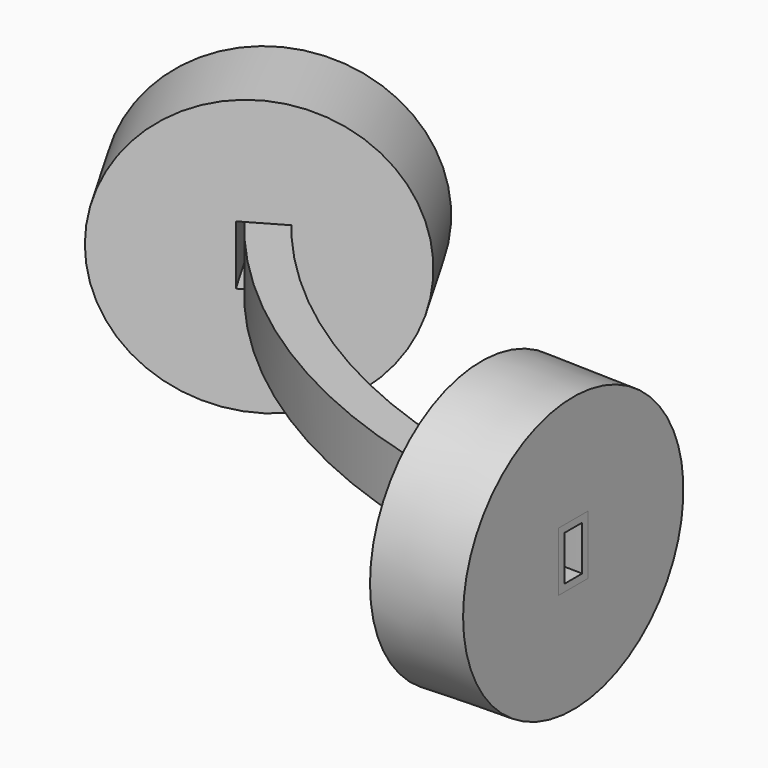
from build123d import *

# Parameters (mm, degrees)
F4_W     = 2.55
F4_H     = 4.1
F4_W_2   = 1.55
F4_H_2   = 3.1
F3_W     = 2.55
F3_H     = 4.1
F3_W_2   = 1.55
F3_H_2   = 3.1
F3_R     = 9.525
F7_DEPTH = 6.35
F4_R     = 9.525
F8_DEPTH = 6.35
F8_TAPER = -1


# Not quite as in the source:
# - a feature of the source that left no trace in its solid (it failed there, or was rolled back) is left out


with BuildPart() as f5:
    # F5: sweep along a path in F0
    with BuildLine(Plane.XY) as f5_path:
        ThreePointArc((-12.7, 21.9970452561), (3.4029547439, 5.8940905122), (25.4, 0))
    # F4 (on line) + F3 (on line) → F5 (sweep)
    with BuildSketch(Plane(origin=(25.4, 0, 0), x_dir=(0, -1, 0), z_dir=(-1, 0, 0))):
        Rectangle(F4_W, F4_H)
        Rectangle(F4_W_2, F4_H_2, mode=Mode.SUBTRACT)
    with BuildSketch(Plane(origin=(-12.7, 21.9970452561, 0), x_dir=(-0.8660254038, -0.5, 0), z_dir=(-0.5, 0.8660254038, 0))):
        Rectangle(F3_W, F3_H)
        Rectangle(F3_W_2, F3_H_2, mode=Mode.SUBTRACT)
    sweep(path=f5_path.line)

    # F4 (on line) → F8 (join)
    with BuildSketch(Plane(origin=(25.4, 0, 0), x_dir=(0, -1, 0), z_dir=(-1, 0, 0))):
        Circle(F4_R)
        Rectangle(F4_W, F4_H, mode=Mode.SUBTRACT)
    extrude(amount=F8_DEPTH, taper=F8_TAPER)


with BuildPart() as f7:
    # F3 (on line) → F7 (new body)
    with BuildSketch(Plane(origin=(-12.7, 21.9970452561, 0), x_dir=(-0.8660254038, -0.5, 0), z_dir=(-0.5, 0.8660254038, 0))):
        Circle(F3_R)
        Rectangle(F3_W, F3_H, mode=Mode.SUBTRACT)
    extrude(amount=-F7_DEPTH)


solid = Compound([f5.part, f7.part])
